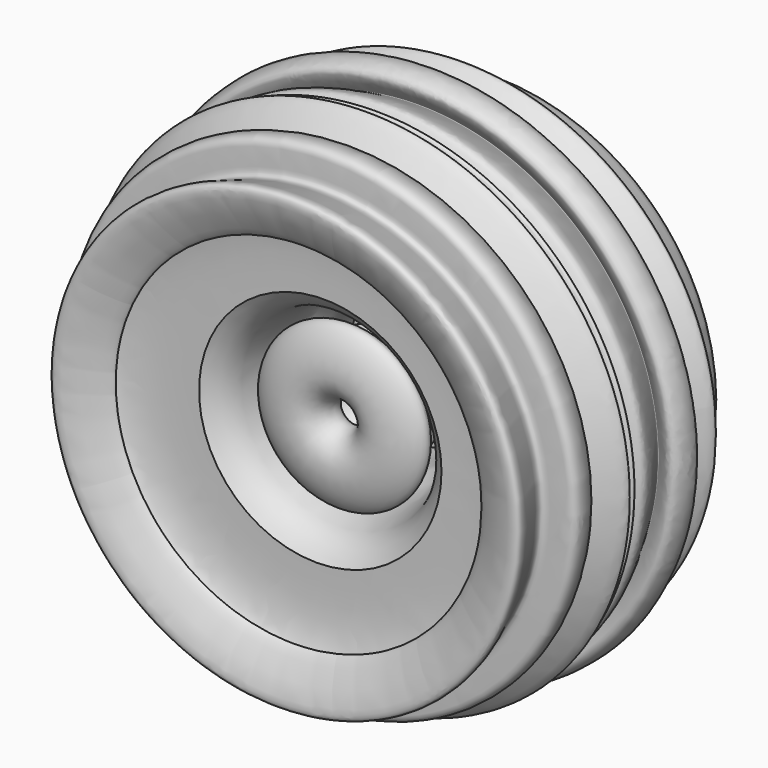
from build123d import *


# Not quite as in the source:
# - a feature of the source that left no trace in its solid (it failed there, or was rolled back) is left out


with BuildPart() as f1:
    # F0 (on Top) → F1 (revolve)
    with BuildSketch(Plane.XY):
        with BuildLine():
            add(Edge.make_bspline(
                [(42.4801555967, 9.2340892239), (44.1352310392, 10.566931445), (51.8187823534, 20.2218648007), (26.3661624451, 30.1922335433), (4.8552341288, 38.6246651057)],
                knots=[0.8366715628, 0.8366715628, 0.8366715628, 0.8366715628, 0.8619543154, 1, 1, 1, 1], degree=3))
            ThreePointArc((4.8552341288, 38.6246651057), (5.6950068631, 72.3647474157), (-14.2162902318, 45.1133507445))
            add(Edge.make_bspline(
                [(-14.2162902318, 45.1133507445), (-16.0527408252, 42.852656592), (-17.8891914185, 40.5919624395), (-19.7256420119, 38.331268287)],
                knots=[0, 0, 0, 0, 8.7378257877, 8.7378257877, 8.7378257877, 8.7378257877], degree=3))
            add(Edge.make_bspline(
                [(-19.7256420119, 38.331268287), (-20.5091562047, 37.5874901911), (-21.2926703976, 36.8437120953), (-22.073547745, 36.1468989247)],
                knots=[0, 0, 0, 0, 0.0427761656, 0.0427761656, 0.0427761656, 0.0427761656], degree=3))
            add(Edge.make_bspline(
                [(-22.073547745, 36.1468989247), (-24.7795924287, 33.569639555), (-27.3324270889, 31.9861436701), (-29.5656006933, 32.4611999126)],
                knots=[0.0429715853, 0.0429715853, 0.0429715853, 0.0429715853, 0.0889245203, 0.0889245203, 0.0889245203, 0.0889245203], degree=3))
            add(Edge.make_bspline(
                [(-29.5656006934, 32.4611999118), (-32.1866168237, 32.867753087), (-34.9610972431, 36.1782498065), (-34.9939843364, 38.9250639476), (-34.9806074249, 39.2097729023)],
                knots=[0.1828177192, 0.1828177192, 0.1828177192, 0.1828177192, 0.3352851245, 0.3535376808, 0.3535376808, 0.3535376808, 0.3535376808], degree=3))
            add(Edge.make_bspline(
                [(-34.9806074241, 39.2097729015), (-35.0153275358, 39.4058165418), (-35.1949177098, 40.8238589515), (-34.7402458735, 41.7692004075), (-35.0868811593, 42.2746760212)],
                knots=[0.1448922732, 0.1448922732, 0.1448922732, 0.1448922732, 0.1492157446, 0.1772429091, 0.1772429091, 0.1772429091, 0.1772429091], degree=3))
            add(Edge.make_bspline(
                [(-35.0868811593, 42.2746760212), (-35.15988711, 42.3632644159), (-35.2489301567, 42.4450679966), (-35.3568010032, 42.5195991993)],
                knots=[0.4355180269, 0.4355180269, 0.4355180269, 0.4355180269, 0.4460695516, 0.4460695516, 0.4460695516, 0.4460695516], degree=3))
            add(Edge.make_bspline(
                [(-35.3568010032, 42.5195991993), (-36.9380984579, 43.4661201744), (-44.1040740647, 42.6357341253), (-46.329598884, 39.166800662)],
                knots=[0.182340058, 0.182340058, 0.182340058, 0.182340058, 0.2498761433, 0.2498761433, 0.2498761433, 0.2498761433], degree=3))
            add(Edge.make_bspline(
                [(-46.3295988811, 39.1668006605), (-48.5810843613, 33.7957881014), (-38.6182961995, 22.5670051735), (-34.1375991688, 19.0500002339)],
                knots=[0.6290128407, 0.6290128407, 0.6290128407, 0.6290128407, 0.890959426, 0.890959426, 0.890959426, 0.890959426], degree=3))
            add(Edge.make_bspline(
                [(-34.1375991702, 19.0500002354), (-32.9334754265, 18.3687025973), (-31.6989127113, 17.8015508692), (-30.4419400924, 17.3305346734)],
                knots=[0.3465774052, 0.3465774052, 0.3465774052, 0.3465774052, 0.3603795495, 0.3603795495, 0.3603795495, 0.3603795495], degree=3))
            add(Edge.make_bspline(
                [(-30.4419400924, 17.3305346734), (-27.6002773682, 16.2656990946), (-24.6440809108, 15.6921981305), (-21.6661202301, 15.401936151)],
                knots=[0.3603795495, 0.3603795495, 0.3603795495, 0.3603795495, 0.3915823285, 0.3915823285, 0.3915823285, 0.3915823285], degree=3))
            add(Edge.make_bspline(
                [(-21.6661202301, 15.401936151), (-17.1401112784, 14.9607858275), (-12.5638291796, 15.1738888123), (-8.2629565737, 15.31069113)],
                knots=[0.3915823285, 0.3915823285, 0.3915823285, 0.3915823285, 0.439005405, 0.439005405, 0.439005405, 0.439005405], degree=3))
            add(Edge.make_bspline(
                [(-8.2629565737, 15.31069113), (-6.5774019725, 15.3643053142), (-4.9341484457, 15.4062002212), (-3.3528003842, 15.3924003243)],
                knots=[0.439005405, 0.439005405, 0.439005405, 0.439005405, 0.4575909787, 0.4575909787, 0.4575909787, 0.4575909787], degree=3))
            add(Edge.make_bspline(
                [(-3.3528003842, 15.3924003243), (1.7997098397, 15.347436087), (11.8974972376, 13.9182247057), (-11.7148205444, 31.6668535799), (14.3484221282, 28.284548677), (17.6707533827, 13.6362347163), (20.7264000974, 9.0255095605)],
                knots=[0.4575909787, 0.4575909787, 0.4575909787, 0.4575909787, 0.5181483986, 0.5936213855, 0.669925761, 0.7404076075, 0.7404076075, 0.7404076075, 0.7404076075], degree=3))
            add(Edge.make_bspline(
                [(20.7264000974, 9.0255095605), (21.9292742503, 7.2104691996), (26.8878470595, 2.2158377978), (37.9947648023, 5.6219770051), (42.4801555967, 9.2340892239)],
                knots=[0.7404076075, 0.7404076075, 0.7404076075, 0.7404076075, 0.7681532206, 0.8366715628, 0.8366715628, 0.8366715628, 0.8366715628], degree=3))
        make_face()
        with BuildLine():
            Line((68.0749574383, -40.4132040932), (61.2648054957, -48.3108013868))
            add(Edge.make_bspline(
                [(84.1211132332, -38.4420980717), (83.0982784553, -37.1499593617), (76.252189647, -30.9302310988), (68.0749574383, -40.4132040932), (61.2648054957, -48.3108013868)],
                knots=[0.8389912848, 0.8389912848, 0.8389912848, 0.8389912848, 0.8659089302, 1, 1, 1, 1], degree=3))
            add(Edge.make_bspline(
                [(68.0749574383, -40.4132040932), (66.7325439708, -26.8228855362), (64.7295528591, -6.5450144225), (73.6344555124, -1.1605258003), (89.8931420356, -7.636490414), (40.2637514497, 25.4799327753), (76.4602319115, 21.659839971), (36.4969355579, 48.2777484214), (77.4165484044, 35.7241759052), (33.537304155, 65.8044508056), (37.449927486, 40.6348284826), (25.6629250296, 50.6097347051), (26.5626088449, 63.0453140853), (46.5514382543, 61.3157332568), (59.5410041395, 68.0753250857), (70.6608524122, 65.9983748029), (70.866113714, 43.8548868579), (96.2686887173, 42.6510124126), (63.4639657473, 17.5631468095), (98.8526616286, 28.0857730323), (94.8170784983, -3.7232845384), (72.5495940879, 19.4042296491), (96.200166396, -12.1181198639), (80.6757339071, -14.140557894), (98.7910472859, -21.3547540918), (79.170272096, -25.0508815265), (101.4987412831, -23.7958319469), (90.4637194011, -33.0897681849), (84.1211132332, -38.4420980717)],
                knots=[0, 0, 0, 0, 0.059183511, 0.0882934728, 0.1129482615, 0.1736997947, 0.2065972032, 0.2547908449, 0.291346369, 0.3444657456, 0.3784264818, 0.4085924015, 0.4395644076, 0.4821076326, 0.5218848391, 0.5511366872, 0.5952593018, 0.6329521941, 0.6782198419, 0.7211296961, 0.7618649576, 0.7970501371, 0.8449425191, 0.8700730853, 0.9008298954, 0.9288046968, 0.9588873013, 1, 1, 1, 1], degree=3))
        make_face()
        with BuildLine():
            add(Edge.make_bspline(
                [(20.7264000974, 9.0255095605), (15.0292076336, 3.8796824347), (4.5347465292, -5.5802388149), (27.2812899813, -11.0922963914), (2.5979121341, -26.7795774335), (55.0281769653, -35.9339628312), (20.4562059768, -4.564609694), (67.0470121813, -5.627403668), (50.2987229623, 4.5027895547), (42.4801555967, 9.2340892239)],
                knots=[0, 0, 0, 0, 0.1381608407, 0.2537140768, 0.3748071143, 0.5473100046, 0.6962018237, 0.8582215054, 1, 1, 1, 1], degree=3))
            add(Edge.make_bspline(
                [(20.7264000974, 9.0255095605), (21.9292742503, 7.2104691996), (26.8878470595, 2.2158377978), (37.9947648023, 5.6219770051), (42.4801555967, 9.2340892239)],
                knots=[0.7404076075, 0.7404076075, 0.7404076075, 0.7404076075, 0.7681532206, 0.8366715628, 0.8366715628, 0.8366715628, 0.8366715628], degree=3))
        make_face()
        with BuildLine():
            add(Edge.make_bspline(
                [(-22.073547745, 36.1468989247), (-24.7795924287, 33.569639555), (-27.3324270889, 31.9861436701), (-29.5656006933, 32.4611999126)],
                knots=[0.0429715853, 0.0429715853, 0.0429715853, 0.0429715853, 0.0889245203, 0.0889245203, 0.0889245203, 0.0889245203], degree=3))
            add(Edge.make_bspline(
                [(-22.073547745, 36.1468989247), (-24.6300012092, 33.8656566145), (-27.1581932072, 32.0877801734), (-29.5656006934, 32.4611999118)],
                knots=[0.0427761656, 0.0427761656, 0.0427761656, 0.0427761656, 0.1828177192, 0.1828177192, 0.1828177192, 0.1828177192], degree=3))
        make_face()
        with BuildLine():
            add(Edge.make_bspline(
                [(-3.3528003848, 15.3924003244), (-3.0039424739, 9.4821235986), (-2.3798320749, -1.0914223775), (9.8931067139, -5.8275678949), (5.4139089476, -21.6389133802), (12.2326431267, -44.9604954136), (32.9737040717, -49.352989693), (51.1817239514, -48.6822421985), (61.2648054957, -48.3108013868)],
                knots=[0, 0, 0, 0, 0.1569327486, 0.2807543047, 0.4304236955, 0.6157921462, 0.7872366603, 1, 1, 1, 1], degree=3))
            add(Edge.make_bspline(
                [(-8.2629565737, 15.31069113), (-6.5774019725, 15.3643053142), (-4.9341484457, 15.4062002212), (-3.3528003842, 15.3924003243)],
                knots=[0.439005405, 0.439005405, 0.439005405, 0.439005405, 0.4575909787, 0.4575909787, 0.4575909787, 0.4575909787], degree=3))
            add(Edge.make_bspline(
                [(-8.2629565737, 15.31069113), (-8.2798740097, 6.7422116683), (-8.308409094, -7.812221626), (2.5456707426, -13.736194193), (5.5318688179, -47.7032639304), (15.4107873955, -54.1655609083), (19.5072013885, -56.845203042)],
                knots=[0, 0, 0, 0, 0.2673773088, 0.4542947943, 0.7737277413, 1, 1, 1, 1], degree=3))
            add(Edge.make_bspline(
                [(19.5072013885, -56.845203042), (36.2277506362, -56.0419091421), (60.2743280984, -54.8866558844), (69.5291138637, -70.7082365188), (37.1197806899, -66.883217145), (93.6002180313, -91.4456411831), (60.991381233, -49.3869995975), (92.1753380127, -59.1583267854), (87.6597643967, -42.9124468004), (84.1211132332, -38.4420980717)],
                knots=[0, 0, 0, 0, 0.1797279524, 0.2584748901, 0.3589190503, 0.5039030619, 0.6370108796, 0.7458656311, 0.8389912848, 0.8389912848, 0.8389912848, 0.8389912848], degree=3))
            add(Edge.make_bspline(
                [(84.1211132332, -38.4420980717), (83.0982784553, -37.1499593617), (76.252189647, -30.9302310988), (68.0749574383, -40.4132040932), (61.2648054957, -48.3108013868)],
                knots=[0.8389912848, 0.8389912848, 0.8389912848, 0.8389912848, 0.8659089302, 1, 1, 1, 1], degree=3))
        make_face()
        with BuildLine():
            add(Edge.make_bspline(
                [(-34.9806074241, 39.2097729015), (-35.0153275358, 39.4058165418), (-35.1949177098, 40.8238589515), (-34.7402458735, 41.7692004075), (-35.0868811593, 42.2746760212)],
                knots=[0.1448922732, 0.1448922732, 0.1448922732, 0.1448922732, 0.1492157446, 0.1772429091, 0.1772429091, 0.1772429091, 0.1772429091], degree=3))
            add(Edge.make_bspline(
                [(-34.9806074241, 39.2097729015), (-34.9205257672, 40.4885274124), (-34.519659523, 41.5863861804), (-35.0868811593, 42.2746760212)],
                knots=[0.3535376808, 0.3535376808, 0.3535376808, 0.3535376808, 0.4355180269, 0.4355180269, 0.4355180269, 0.4355180269], degree=3))
        make_face()
        with BuildLine():
            add(Edge.make_bspline(
                [(-21.6661202301, 15.401936151), (-23.2838230452, 12.9028918362), (-26.7489465106, 7.6627062626), (-13.2647443736, 0.2622475452), (-26.4253227572, -7.2214017242), (-8.26604684, -15.0299120026), (-23.7600688777, -21.9122337329), (-17.8653734993, -26.9226639295), (-14.9352010339, -29.4131990522)],
                knots=[0, 0, 0, 0, 0.1531350806, 0.3295821667, 0.4842195754, 0.6682743584, 0.8355343291, 1, 1, 1, 1], degree=3))
            add(Edge.make_bspline(
                [(-30.4419400924, 17.3305346734), (-27.6002773682, 16.2656990946), (-24.6440809108, 15.6921981305), (-21.6661202301, 15.401936151)],
                knots=[0.3603795495, 0.3603795495, 0.3603795495, 0.3603795495, 0.3915823285, 0.3915823285, 0.3915823285, 0.3915823285], degree=3))
            add(Edge.make_bspline(
                [(-30.4419400924, 17.3305346734), (-31.9925919804, 14.0306384674), (-35.1336354416, 7.3389782371), (-19.3266845089, -0.4456044084), (-37.3297607575, -4.3478989021), (-21.3218384605, -12.8871572079), (-34.9111018779, -19.5270932251), (-28.9992347505, -25.4183546163), (-25.9080007672, -28.4988004714)],
                knots=[0, 0, 0, 0, 0.168823053, 0.3430307564, 0.500449518, 0.6670616803, 0.8259557189, 1, 1, 1, 1], degree=3))
            add(Edge.make_bspline(
                [(-25.9080007672, -28.4988004714), (-30.7442998208, -30.2962020187), (-41.2643252435, -34.2059498987), (-28.5264937866, -58.2564239002), (10.9656465408, -42.1376706897), (-6.804654615, -33.4075435232), (-14.9352010339, -29.4131990522)],
                knots=[0, 0, 0, 0, 0.2066536181, 0.4495175529, 0.7481346518, 1, 1, 1, 1], degree=3))
        make_face()
        with BuildLine():
            add(Edge.make_bspline(
                [(-35.3568010032, 42.5195991993), (-36.9380984579, 43.4661201744), (-44.1040740647, 42.6357341253), (-46.329598884, 39.166800662)],
                knots=[0.182340058, 0.182340058, 0.182340058, 0.182340058, 0.2498761433, 0.2498761433, 0.2498761433, 0.2498761433], degree=3))
            add(Edge.make_bspline(
                [(-35.3568010032, 42.5195991993), (-37.2270754895, 43.8118279278), (-44.7571631868, 42.9179116211), (-46.3295988811, 39.1668006605)],
                knots=[0.4460695516, 0.4460695516, 0.4460695516, 0.4460695516, 0.6290128407, 0.6290128407, 0.6290128407, 0.6290128407], degree=3))
        make_face()
        with BuildLine():
            add(Edge.make_bspline(
                [(-34.1375991702, 19.0500002354), (-32.2724182356, 17.5859756613), (-31.357179164, 17.4582551673), (-30.4419400924, 17.3305346734)],
                knots=[0.890959426, 0.890959426, 0.890959426, 0.890959426, 1, 1, 1, 1], degree=3))
            add(Edge.make_bspline(
                [(-34.1375991702, 19.0500002354), (-32.9334754265, 18.3687025973), (-31.6989127113, 17.8015508692), (-30.4419400924, 17.3305346734)],
                knots=[0.3465774052, 0.3465774052, 0.3465774052, 0.3465774052, 0.3603795495, 0.3603795495, 0.3603795495, 0.3603795495], degree=3))
        make_face()
    revolve(axis=Axis((-44.6120854467, -10.7344947755, 0), (0.0451285099, -0.9989811898, 0)))


solid = f1.part
